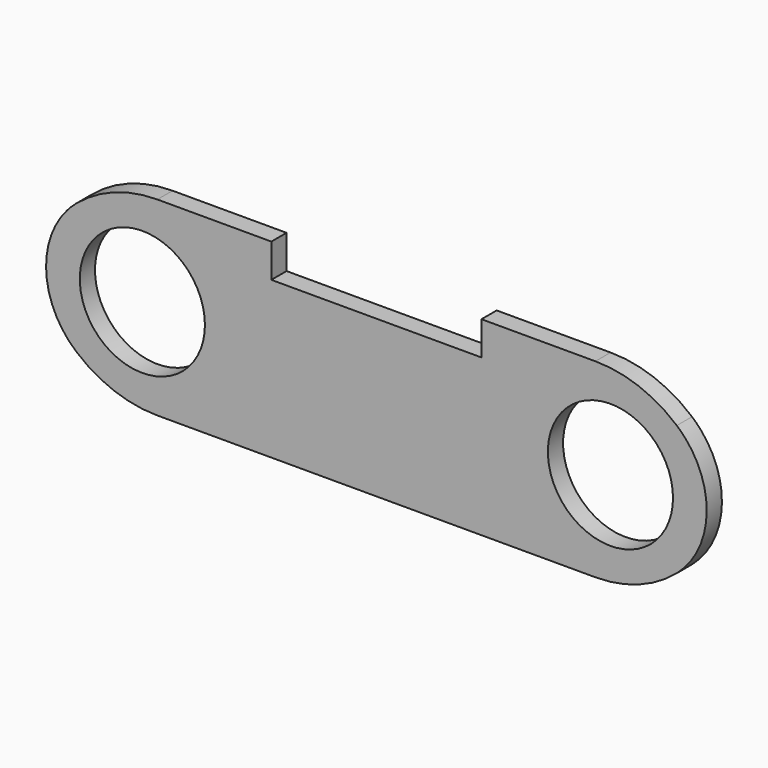
from build123d import *

# Parameters (mm, degrees)
F0_R        = 16.7132
F1_DEPTH    = 5.08
F2_T1_DEPTH = 172.212
F3_R        = 22.86
F4_R        = 22.86


# Not quite as in the source:
# - a fillet or chamfer that OpenCascade refuses, or shapes differently, is made with other operations: its cross-section is extruded or revolved along the edge and cut away or added


with BuildPart() as f1:
    # F0 (on Front) → F1 (new body)
    with BuildSketch(Plane.XZ):
        Polygon((-91.9353, -25.4), (91.9353, -25.4), (91.9353, 25.4), (28.067, 25.4), (28.067, 16.4), (-28.067, 16.4), (-28.067, 25.4), (-91.9353, 25.4), align=None)
        with Locations((-62.5221, 0)):
            Circle(F0_R, mode=Mode.SUBTRACT)
        with Locations((62.5221, 0)):
            Circle(F0_R, mode=Mode.SUBTRACT)
    extrude(amount=F1_DEPTH)

    # F2: fillet of radius 33.4264 on 4 edges, made by hand

    # F2_s2 → F2_t1 (cut)
    with BuildSketch(Plane.XZ.offset(-83.566)):
        with BuildLine():
            ThreePointArc((91.9353, -8.0264), (82.1449341107, 15.6096341107), (58.5089, 25.4))
            Line((58.5089, 25.4), (91.9353, 25.4))
            Line((91.9353, 25.4), (91.9353, -8.0264))
        make_face()
        with BuildLine():
            ThreePointArc((58.5089, -25.4), (82.1449341107, -15.6096341107), (91.9353, 8.0264))
            Line((91.9353, 8.0264), (91.9353, -25.4))
            Line((91.9353, -25.4), (58.5089, -25.4))
        make_face()
        with BuildLine():
            ThreePointArc((-58.5089, 25.4), (-82.1449341107, 15.6096341107), (-91.9353, -8.0264))
            Line((-91.9353, -8.0264), (-91.9353, 25.4))
            Line((-91.9353, 25.4), (-58.5089, 25.4))
        make_face()
        with BuildLine():
            ThreePointArc((-91.9353, 8.0264), (-82.1449341107, -15.6096341107), (-58.5089, -25.4))
            Line((-58.5089, -25.4), (-91.9353, -25.4))
            Line((-91.9353, -25.4), (-91.9353, 8.0264))
        make_face()
    extrude(amount=F2_T1_DEPTH, mode=Mode.SUBTRACT)

    # F3
    f3_edges = [f1.edges().sort_by_distance(p)[0] for p in [
        (-90.957338, -2.54, 0),
    ]]
    fillet(f3_edges, radius=F3_R)

    # F4
    f4_edges = [f1.edges().sort_by_distance(p)[0] for p in [
        (90.957338, -2.54, 0),
    ]]
    fillet(f4_edges, radius=F4_R)


solid = f1.part
